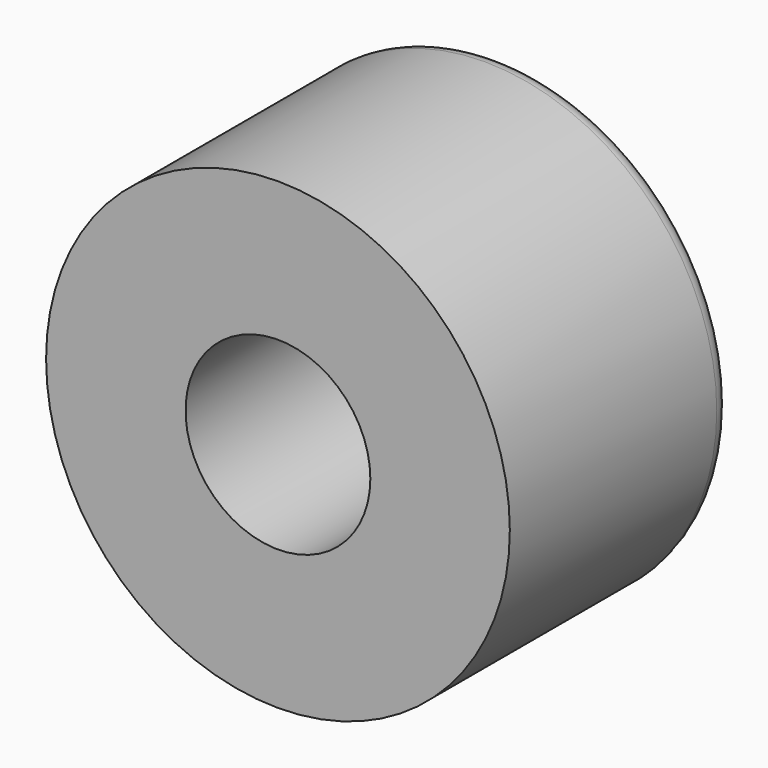
from build123d import *

# Parameters (mm, degrees)
F0_R           = 25.1
F1_DEPTH       = 30
F2_R           = 2
F5_D           = 20
F5_DEPTH       = 190
F5_CSINK_D     = 22
F5_CSINK_ANGLE = 90
F5_TIP         = 6.0086061903


# Not quite as in the source:
# - a feature of the source that left no trace in its solid (it failed there, or was rolled back) is left out


with BuildPart() as f1:
    # F0 (on Front) → F1 (new body)
    with BuildSketch(Plane.XZ):
        with Locations((20.5169470484, 0)):
            Circle(F0_R)
    extrude(amount=F1_DEPTH)

    # F2
    f2_edges = [f1.edges().sort_by_distance(p)[0] for p in [
        (-4.583053, 0, 0),
    ]]
    fillet(f2_edges, radius=F2_R)

    # F5
    with Locations(Plane(origin=(0, 0, 0), x_dir=(-1, 0, 0), z_dir=(0, 1, 0))):
        with Locations((-20.5169470484, 0)):
            CounterSinkHole(F5_D / 2, F5_CSINK_D / 2, depth=F5_DEPTH, counter_sink_angle=F5_CSINK_ANGLE)
            with Locations((0, 0, -(F5_DEPTH + F5_TIP / 2))):  # 118° drill point
                Cone(0, F5_D / 2, F5_TIP, mode=Mode.SUBTRACT)


solid = f1.part
